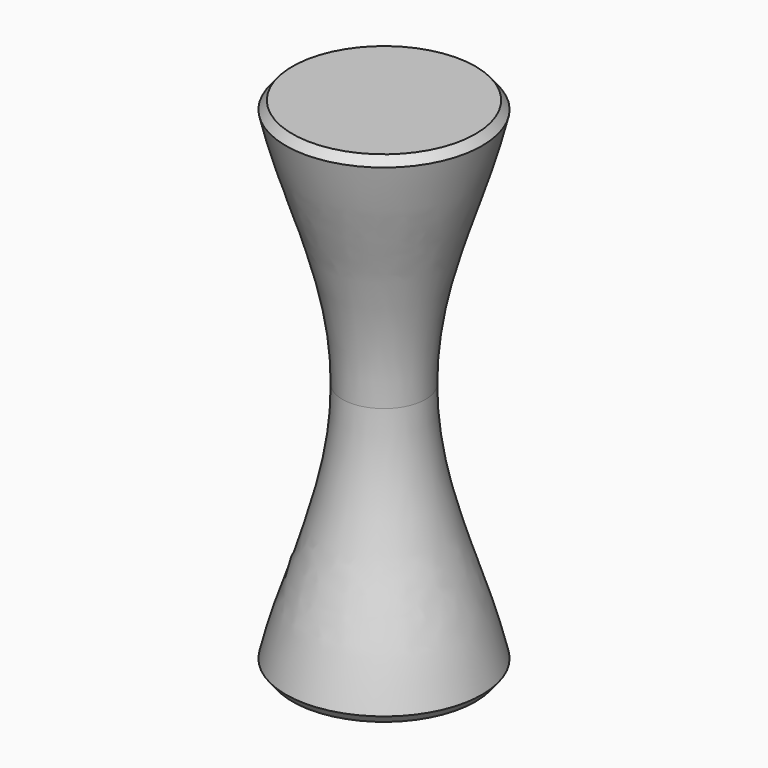
from build123d import *


# Not quite as in the source:
# - a fillet or chamfer that OpenCascade refuses, or shapes differently, is made with other operations: its cross-section is extruded or revolved along the edge and cut away or added


with BuildPart() as f1:
    # F0 (on Front) → F1 (revolve)
    with BuildSketch(Plane.XZ):
        with BuildLine():
            Line((0, 0), (0, -30))
            Line((0, -30), (12, -30))
            add(Edge.make_bspline(
                [(5, 0), (5, -11.6286956261), (9.7787035629, -19.5170734078), (12, -30)],
                knots=[0, 0, 0, 0, 30.8058436015, 30.8058436015, 30.8058436015, 30.8058436015], degree=3))
            Line((5, 0), (0, 0))
        make_face()
    revolve(axis=Axis((0, 0, -15), (0, 0, -1)))

    # F2: chamfer of 1 on 1 edges, made by hand

    # F2_s1 → F2_t2 (revolve, cut)
    with BuildSketch(Plane.XZ):
        with BuildLine():
            Line((10.966073896, -30.0312962065), (11.8055530365, -28.9766322442))
            Line((11.8055530365, -28.9766322442), (11.8250433673, -28.9721459307))
            ThreePointArc((11.8250433673, -28.9721459307), (11.9092913241, -29.4868738611), (12.0195655741, -29.9958541215))
            Line((12.0195655741, -29.9958541215), (12, -30.02))
            ThreePointArc((12, -30.02), (11.483036948, -30.02), (10.966073896, -30.0512962065))
            Line((10.966073896, -30.0512962065), (10.966073896, -30.0312962065))
        make_face()
    revolve(axis=Axis((0, 0, -30), (0, 0, -1)), mode=Mode.SUBTRACT)

    # F3: F1 across plane


with BuildPart() as f1_1:
    add(f1.part)
    add(f1.part.mirror(Plane.XY))


solid = f1_1.part
